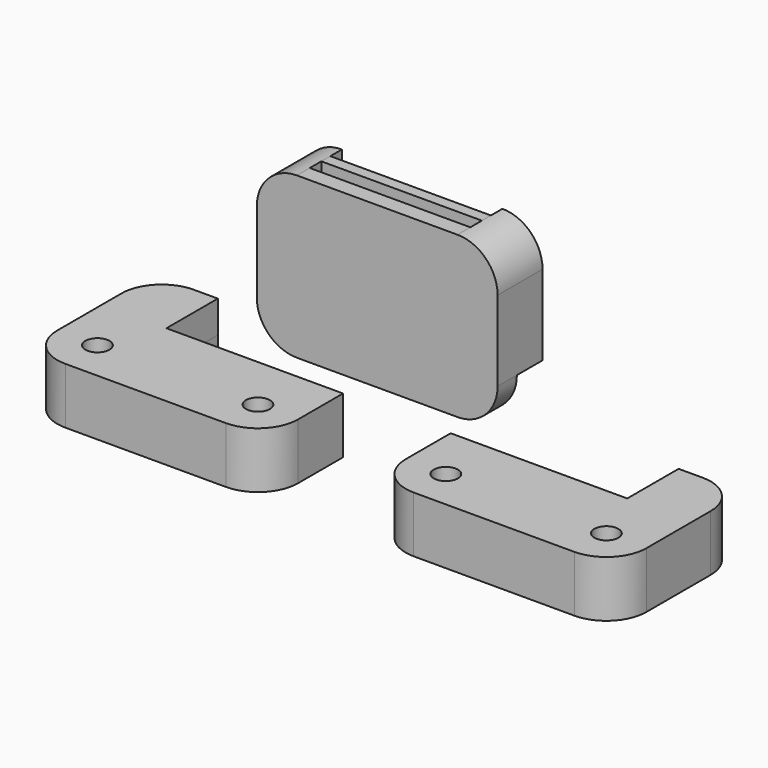
from build123d import *

# Parameters (mm, degrees)
F0_R          = 1.5
F1_DEPTH      = 4
F2_DEPTH      = 3
F3_T4_DEPTH   = 54.3417857624
F3_2_T4_DEPTH = 54.3417857624
F4_SIZE       = 2
F4_2_SIZE     = 2
F5_DEPTH      = 10
F0_W          = 20
F0_H          = 1.8
F0_H_2        = 0.8
F6_DEPTH      = 5
F0_H_3        = 1
F7_DEPTH      = 10
F8_R          = 4.99999


# Not quite as in the source:
# - a fillet or chamfer that OpenCascade refuses, or shapes differently, is made with other operations: its cross-section is extruded or revolved along the edge and cut away or added
# - a fillet or chamfer is up to 0.001 mm smaller than in the source, because OpenCascade refuses the exact size


with BuildPart() as f1:
    # F0 (on Top) → F1 (new body)
    with BuildSketch(Plane.XY):
        with BuildLine():
            Line((5.2090043873, -15.0646343827), (2.2090043873, -15.0646343827))
            ThreePointArc((2.2090043873, -15.0646343827), (-1.3265295187, -16.5291004768), (-2.7909956127, -20.0646343827))
            Line((-2.7909956127, -20.0646343827), (-2.7909956127, -30.0646343827))
            ThreePointArc((-2.7909956127, -30.0646343827), (-1.3265295187, -33.6001682887), (2.2090043873, -35.0646343827))
            Line((2.2090043873, -35.0646343827), (22.2090043873, -35.0646343827))
            ThreePointArc((22.2090043873, -35.0646343827), (25.7445382932, -33.6001682887), (27.2090043873, -30.0646343827))
            Line((27.2090043873, -30.0646343827), (27.2090043873, -23.0646343827))
            Line((27.2090043873, -23.0646343827), (5.2090043873, -23.0646343827))
            Line((5.2090043873, -23.0646343827), (5.2090043873, -15.0646343827))
        make_face()
        with Locations((2.2090043873, -30.0646343827)):
            Circle(F0_R, mode=Mode.SUBTRACT)
        with Locations((22.2090043873, -30.0646343827)):
            Circle(F0_R, mode=Mode.SUBTRACT)
    extrude(amount=F1_DEPTH)

    # F0 (on Top) → F2 (join)
    with BuildSketch(Plane.XY):
        Polygon((27.2090043873, -23.0646343827), (5.2090043873, -15.0646343827), (5.2090043873, -23.0646343827), align=None)
        with BuildLine():
            Line((5.2090043873, -15.0646343827), (2.2090043873, -15.0646343827))
            ThreePointArc((2.2090043873, -15.0646343827), (-1.3265295187, -16.5291004768), (-2.7909956127, -20.0646343827))
            Line((-2.7909956127, -20.0646343827), (-2.7909956127, -30.0646343827))
            ThreePointArc((-2.7909956127, -30.0646343827), (-1.3265295187, -33.6001682887), (2.2090043873, -35.0646343827))
            Line((2.2090043873, -35.0646343827), (22.2090043873, -35.0646343827))
            ThreePointArc((22.2090043873, -35.0646343827), (25.7445382932, -33.6001682887), (27.2090043873, -30.0646343827))
            Line((27.2090043873, -30.0646343827), (27.2090043873, -23.0646343827))
            Line((27.2090043873, -23.0646343827), (5.2090043873, -23.0646343827))
            Line((5.2090043873, -23.0646343827), (5.2090043873, -15.0646343827))
        make_face()
        with Locations((2.2090043873, -30.0646343827)):
            Circle(F0_R, mode=Mode.SUBTRACT)
        with Locations((22.2090043873, -30.0646343827)):
            Circle(F0_R, mode=Mode.SUBTRACT)
    extrude(amount=-F2_DEPTH)

    # F3: fillet of radius 5 on 1 edges, made by hand


with BuildPart() as f1b:
    # F0 (on Top) → F1, piece 2 (new body)
    with BuildSketch(Plane.XY):
        with BuildLine():
            Line((65.6200699508, -15.0646343827), (62.6200699508, -15.0646343827))
            Line((62.6200699508, -15.0646343827), (62.6200699508, -23.0646343827))
            Line((62.6200699508, -23.0646343827), (40.6200699508, -23.0646343827))
            Line((40.6200699508, -23.0646343827), (40.6200699508, -30.0646343827))
            ThreePointArc((40.6200699508, -30.0646343827), (42.0845360449, -33.6001682887), (45.6200699508, -35.0646343827))
            Line((45.6200699508, -35.0646343827), (65.6200699508, -35.0646343827))
            ThreePointArc((65.6200699508, -35.0646343827), (69.1556038568, -33.6001682887), (70.6200699508, -30.0646343827))
            Line((70.6200699508, -30.0646343827), (70.6200699508, -20.0646343827))
            ThreePointArc((70.6200699508, -20.0646343827), (69.1556038568, -16.5291004768), (65.6200699508, -15.0646343827))
        make_face()
        with Locations((45.6200699508, -30.0646343827)):
            Circle(F0_R, mode=Mode.SUBTRACT)
        with Locations((65.6200699508, -30.0646343827)):
            Circle(F0_R, mode=Mode.SUBTRACT)
    extrude(amount=F1_DEPTH)

    # F0 (on Top) → F2, piece 2 (join)
    with BuildSketch(Plane.XY):
        with BuildLine():
            Line((65.6200699508, -15.0646343827), (62.6200699508, -15.0646343827))
            Line((62.6200699508, -15.0646343827), (62.6200699508, -23.0646343827))
            Line((62.6200699508, -23.0646343827), (40.6200699508, -23.0646343827))
            Line((40.6200699508, -23.0646343827), (40.6200699508, -30.0646343827))
            ThreePointArc((40.6200699508, -30.0646343827), (42.0845360449, -33.6001682887), (45.6200699508, -35.0646343827))
            Line((45.6200699508, -35.0646343827), (65.6200699508, -35.0646343827))
            ThreePointArc((65.6200699508, -35.0646343827), (69.1556038568, -33.6001682887), (70.6200699508, -30.0646343827))
            Line((70.6200699508, -30.0646343827), (70.6200699508, -20.0646343827))
            ThreePointArc((70.6200699508, -20.0646343827), (69.1556038568, -16.5291004768), (65.6200699508, -15.0646343827))
        make_face()
        with Locations((45.6200699508, -30.0646343827)):
            Circle(F0_R, mode=Mode.SUBTRACT)
        with Locations((65.6200699508, -30.0646343827)):
            Circle(F0_R, mode=Mode.SUBTRACT)
        Polygon((62.6200699508, -23.0646343827), (62.6200699508, -15.0646343827), (40.6200699508, -23.0646343827), align=None)
    extrude(amount=-F2_DEPTH)

    # F3#2: fillet of radius 5 on 1 edges, made by hand


with BuildPart() as f3_tool2:
    # F3_s3 → F3_t4 (new body)
    with BuildSketch(Plane(origin=(42.2056164979, -15.3474969083, 0), x_dir=(0, 0, 1), z_dir=(-0.9397934235, 0.3417430631, 0))):
        with BuildLine():
            ThreePointArc((0, -16.9600789002), (-0.8166998673, -14.2214661126), (-3, -12.3775032052))
            Line((-3, -12.3775032052), (0, -12.3775032052))
            Line((0, -12.3775032052), (0, -16.9600789002))
        make_face()
    extrude(amount=F3_T4_DEPTH)

    split(bisect_by=Plane.XZ.offset(23.0646343827), keep=Keep.BOTTOM)

    split(bisect_by=Plane.YZ.offset(5.2090043873), keep=Keep.TOP)


with BuildPart() as f1_1:
    add(f1.part)

    # F3_t1: cut F3_tool2
    add(f3_tool2.part, mode=Mode.SUBTRACT)

    # F4
    f4_edges = [f1_1.edges().sort_by_distance(p)[0] for p in [
        (20.709004, -30.064634, -3),
        (0.709004, -30.064634, -3),
    ]]
    chamfer(f4_edges, length=F4_SIZE)


with BuildPart() as f3_2_tool2:
    # F3_2_s3 → F3_2_t4 (new body)
    with BuildSketch(Plane(origin=(68.771867002, 25.0079516371, 0), x_dir=(0, 0, 1), z_dir=(-0.9397934235, -0.3417430631, 0))):
        with BuildLine():
            ThreePointArc((0, -40.1401945308), (-0.8166998673, -37.4015817433), (-3, -35.5576188358))
            Line((-3, -35.5576188358), (0, -35.5576188358))
            Line((0, -35.5576188358), (0, -40.1401945308))
        make_face()
    extrude(amount=F3_2_T4_DEPTH)

    split(bisect_by=Plane.XZ.offset(23.0646343827), keep=Keep.BOTTOM)

    split(bisect_by=Plane.YZ.offset(62.6200699508), keep=Keep.BOTTOM)


with BuildPart() as f1b_1:
    add(f1b.part)

    # F3_2_t1: cut F3_2_tool2
    add(f3_2_tool2.part, mode=Mode.SUBTRACT)

    # F4#2
    f4_2_edges = [f1b_1.edges().sort_by_distance(p)[0] for p in [
        (64.12007, -30.064634, -3),
        (44.12007, -30.064634, -3),
    ]]
    chamfer(f4_2_edges, length=F4_2_SIZE)


with BuildPart() as f5:
    # F0 (on Top) → F5 (new body)
    with BuildSketch(Plane.XY):
        Polygon((2.2090043873, 8.0083264206), (-2.7909956127, 8.0083264206), (-2.7909956127, 4.0083264206), (2.2090043873, 4.0083264206), (2.2090043873, 4.8083264206), (22.2090043873, 4.8083264206), (22.2090043873, 4.0083264206), (27.2090043873, 4.0083264206), (27.2090043873, 8.0083264206), (22.2090043873, 8.0083264206), (22.2090043873, 6.2083264206), (2.2090043873, 6.2083264206), align=None)
        Polygon((2.2090043873, 4.0083264206), (-2.7909956127, 4.0083264206), (-2.7909956127, 1.0083264206), (27.2090043873, 1.0083264206), (27.2090043873, 4.0083264206), (22.2090043873, 4.0083264206), (22.2090043873, 3.0083264206), (2.2090043873, 3.0083264206), align=None)
    extrude(amount=F5_DEPTH)

    # F0 (on Top) → F6 (join)
    with BuildSketch(Plane.XY):
        Polygon((2.2090043873, 8.0083264206), (-2.7909956127, 8.0083264206), (-2.7909956127, 4.0083264206), (2.2090043873, 4.0083264206), (2.2090043873, 4.8083264206), (22.2090043873, 4.8083264206), (22.2090043873, 4.0083264206), (27.2090043873, 4.0083264206), (27.2090043873, 8.0083264206), (22.2090043873, 8.0083264206), (22.2090043873, 6.2083264206), (2.2090043873, 6.2083264206), align=None)
        with Locations((12.2090043873, 7.1083264206)):
            Rectangle(F0_W, F0_H)
        Polygon((2.2090043873, 4.0083264206), (-2.7909956127, 4.0083264206), (-2.7909956127, 1.0083264206), (27.2090043873, 1.0083264206), (27.2090043873, 4.0083264206), (22.2090043873, 4.0083264206), (22.2090043873, 3.0083264206), (2.2090043873, 3.0083264206), align=None)
        with Locations((12.2090043873, 4.4083264206)):
            Rectangle(F0_W, F0_H_2)
    extrude(amount=-F6_DEPTH)

    # F0 (on Top) → F7 (join)
    with BuildSketch(Plane.XY):
        Polygon((2.2090043873, 4.0083264206), (-2.7909956127, 4.0083264206), (-2.7909956127, 1.0083264206), (27.2090043873, 1.0083264206), (27.2090043873, 4.0083264206), (22.2090043873, 4.0083264206), (22.2090043873, 3.0083264206), (2.2090043873, 3.0083264206), align=None)
        with Locations((12.2090043873, 3.5083264206)):
            Rectangle(F0_W, F0_H_3)
    extrude(amount=-F7_DEPTH)

    # F8 (radius 5 in the source; OpenCascade refuses exactly that, so slightly less here)
    f8_edges = [f5.edges().sort_by_distance(p)[0] for p in [
        (-2.790996, 4.508326, 10),
        (27.209004, 4.508326, 10),
        (27.209004, 2.508326, -10),
        (-2.790996, 2.508326, -10),
    ]]
    fillet(f8_edges, radius=F8_R)


solid = Compound([f1_1.part, f1b_1.part, f5.part])
